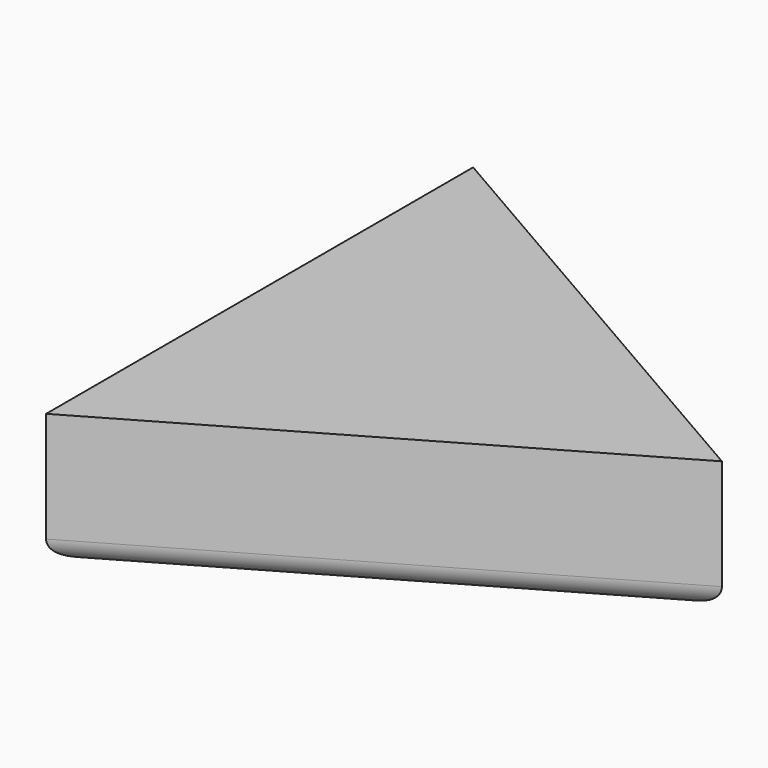
from build123d import *

# Parameters (mm, degrees)
F1_DEPTH    = 29.464
F2_R        = 23.506947033
F3_DEPTH    = 36.322
F4_SIZE     = 5.08
F5_T3_DEPTH = 143.4285494589
F5_T5_DEPTH = 137.562670724
F5_T7_DEPTH = 131.696791989
F6_SIZE     = 5.08
F7_SIZE     = 5.08
F8_SIZE     = 5.08


# Not quite as in the source:
# - a fillet or chamfer that OpenCascade refuses, or shapes differently, is made with other operations: its cross-section is extruded or revolved along the edge and cut away or added


with BuildPart() as f1:
    # F0 (on Top) → F1 (new body)
    with BuildSketch(Plane.XY):
        Polygon((-34.0719074011, 59.0142747295), (-34.0719074011, -59.0142747295), (68.1438148022, 0), align=None)
    extrude(amount=F1_DEPTH)

    # F2 (on face) → F3 (join)
    with BuildSketch(Plane.XY.offset(29.464)):
        Circle(F2_R)
    extrude(amount=-F3_DEPTH)

    # F4
    f4_edges = [f1.edges().sort_by_distance(p)[0] for p in [
        (-23.506947, 0, -6.858),
    ]]
    chamfer(f4_edges, length=F4_SIZE)

    # F5: fillet of radius 5.08 on 4 edges, made by hand

    # F5_s1 → F5_t2 (revolve)
    with BuildSketch(Plane.XZ):
        with BuildLine():
            ThreePointArc((23.506947033, -1.778), (25.2422963406, -0.4658608604), (27.367412808, 0))
            Line((27.367412808, 0), (23.506947033, 0))
            Line((23.506947033, 0), (23.506947033, -1.778))
        make_face()
    revolve(axis=Axis((0, 0, 0), (0, 0, 1)))

    # F5_s4 → F5_t3 (cut)
    with BuildSketch(Plane(origin=(62.1063837297, -35.8571373647, 0), x_dir=(0, 0, 1), z_dir=(-0.8660254038, 0.5, 0))):
        with BuildLine():
            ThreePointArc((0, 28.9919074011), (1.4878975516, 32.5840098495), (5.08, 34.0719074011))
            Line((5.08, 34.0719074011), (0, 34.0719074011))
            Line((0, 34.0719074011), (0, 28.9919074011))
        make_face()
    extrude(amount=F5_T3_DEPTH, mode=Mode.SUBTRACT)

    # F5_s6 → F5_t5 (cut)
    with BuildSketch(Plane(origin=(-62.1063837297, -35.8571373647, 0), x_dir=(0, 0, 1), z_dir=(0.8660254038, 0.5, 0))):
        with BuildLine():
            ThreePointArc((0, 28.9919074011), (1.4878975516, 32.5840098495), (5.08, 34.0719074011))
            Line((5.08, 34.0719074011), (0, 34.0719074011))
            Line((0, 34.0719074011), (0, 28.9919074011))
        make_face()
    extrude(amount=F5_T5_DEPTH, mode=Mode.SUBTRACT)

    # F5_s8 → F5_t7 (cut)
    with BuildSketch(Plane.XZ.offset(-65.8483959945)):
        with BuildLine():
            ThreePointArc((-28.9919074011, 0), (-32.5840098495, 1.4878975516), (-34.0719074011, 5.08))
            Line((-34.0719074011, 5.08), (-34.0719074011, 0))
            Line((-34.0719074011, 0), (-28.9919074011, 0))
        make_face()
    extrude(amount=F5_T7_DEPTH, mode=Mode.SUBTRACT)

    # F6
    f6_edges = [f1.edges().sort_by_distance(p)[0] for p in [
        (-18.426947, 0, -6.858),
    ]]
    chamfer(f6_edges, length=F6_SIZE)

    # F7
    f7_edges = [f1.edges().sort_by_distance(p)[0] for p in [
        (-13.346947, 0, -6.858),
    ]]
    chamfer(f7_edges, length=F7_SIZE)

    # F8
    f8_edges = [f1.edges().sort_by_distance(p)[0] for p in [
        (-8.266947, 0, -6.858),
    ]]
    chamfer(f8_edges, length=F8_SIZE)


solid = f1.part
